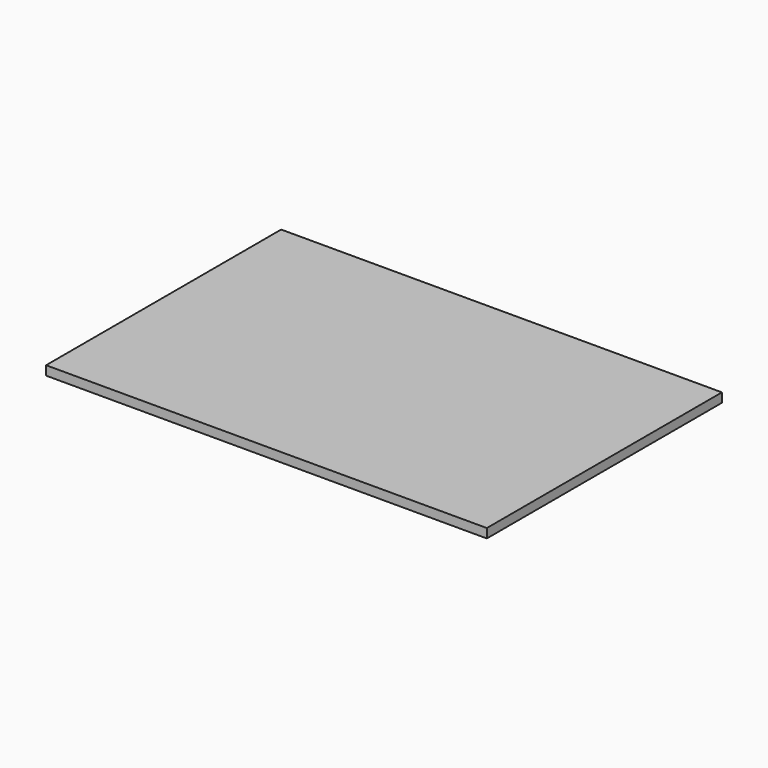
from build123d import *

# Parameters (mm, degrees)
F0_W     = 1200
F0_H     = 800
F1_DEPTH = 25


# Not quite as in the source:
# - the program builds the solid bodies; features that only make, move or delete a surface that nothing else refers to are left out


with BuildPart() as f1:
    # F0 (on Top) → F1 (new body)
    with BuildSketch(Plane.XY):
        with Locations((-600, 400)):
            Rectangle(F0_W, F0_H)
    extrude(amount=F1_DEPTH)


solid = f1.part
